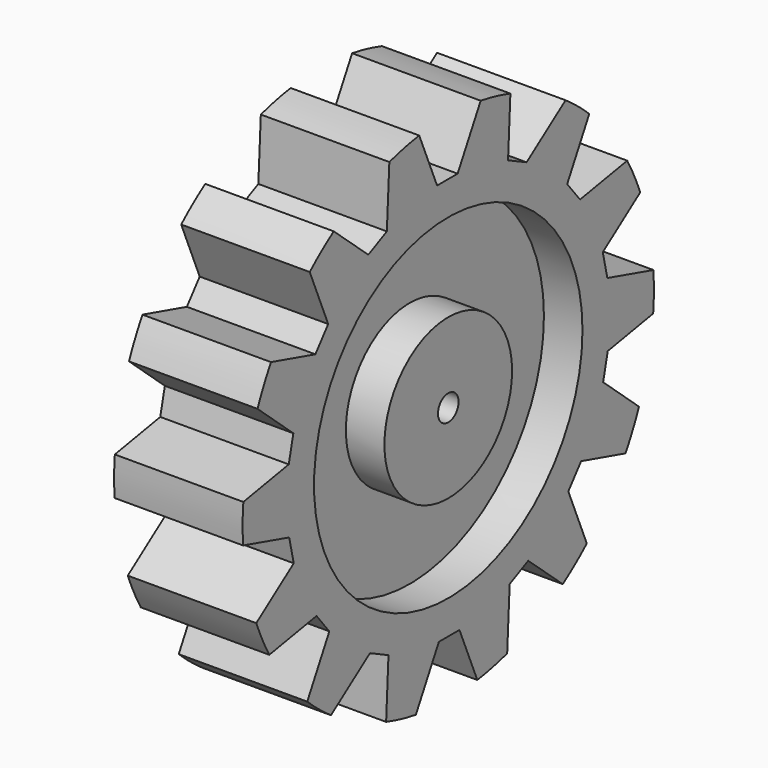
from build123d import *

# Parameters (mm, degrees)
F0_R            = 50.8
F1_DEPTH        = 25.4
F3_DEPTH        = 76.2
F3_COPIES_COUNT = 14
F5_R            = 33.1589866973
F6_DEPTH        = 7.62
F7_R            = 15.7705666828
F8_DEPTH        = 7.62
F9_R            = 2.54
F10_DEPTH       = 76.2


# Not quite as in the source:
# - a feature of the source that left no trace in its solid (it failed there, or was rolled back) is left out
# - a pattern or mirror of a feature is missing from the dataset's text; its kind, count and spacing are read off the source's solid


with BuildPart() as f1:
    # F0 (on Right) → F1 (new body)
    with BuildSketch(Plane.YZ):
        Circle(F0_R)
    extrude(amount=F1_DEPTH)

    # F2 (on face) → F3 (cut)
    with BuildSketch(Plane.YZ.offset(25.4)):
        with BuildLine():
            Line((2.3186472245, 39.7838875651), (8.0035195906, 50.1655626318))
            ThreePointArc((8.0035195906, 50.1655626318), (0.4157775456, 50.7982984856), (-7.181304959, 50.2898484695))
            Line((-7.181304959, 50.2898484695), (-2.7636629529, 39.7838875651))
            Line((-2.7636629529, 39.7838875651), (2.3186472245, 39.7838875651))
        make_face()
    f3 = extrude(amount=-F3_DEPTH, mode=Mode.SUBTRACT)

    # F3_copies: F3 ×14 about axis
    f3_copies_axis = Axis((0, 0, 0), (1, 0, 0))
    for i in range(1, F3_COPIES_COUNT):
        add(f3.rotate(f3_copies_axis, i * 360 / F3_COPIES_COUNT), mode=Mode.SUBTRACT)

    # F5 (on face) → F6 (cut)
    with BuildSketch(Plane.YZ.offset(25.4)):
        Circle(F5_R)
    extrude(amount=-F6_DEPTH, mode=Mode.SUBTRACT)

    # F7 (on face) → F8 (join)
    with BuildSketch(Plane.YZ.offset(17.78)):
        Circle(F7_R)
    extrude(amount=F8_DEPTH)

    # F9 (on face) → F10 (cut)
    with BuildSketch(Plane.YZ.offset(25.4)):
        Circle(F9_R)
    extrude(amount=-F10_DEPTH, mode=Mode.SUBTRACT)


solid = f1.part
